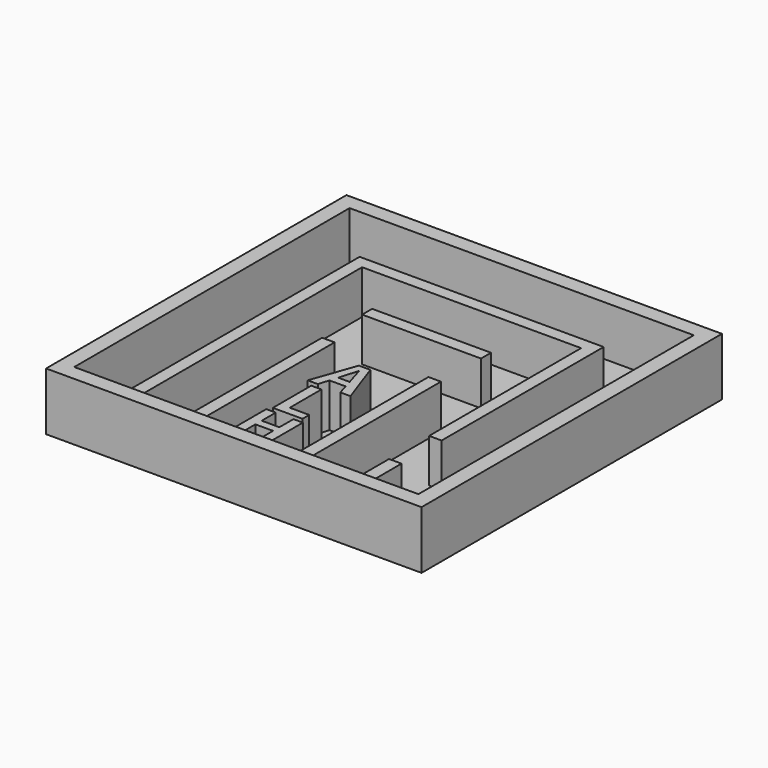
from build123d import *

# Parameters (mm, degrees)
F0_W          = 38.1
F0_H          = 38.1
F1_DEPTH      = 0.79375
F2_W          = 38.1
F2_H          = 38.1
F2_W_2        = 34.925
F2_H_2        = 34.925
F3_DEPTH      = 5.08
F4_W          = 12.065
F4_H          = 1.27
F4_W_2        = 1.27
F4_H_2        = 17.145
F4_H_3        = 4.210835259
F5_DEPTH      = 4.445
F4_R          = 1.27
F6_DEPTH      = 0.396875
F7_TEXT_SIZE  = 6.295947565
F8_DEPTH      = 4.445
F9_TEXT_SIZE  = 6.8291077494
F10_TEXT_SIZE = 6.3526599358
F11_DEPTH     = 4.445


# Not quite as in the source:
# - Text() gives the source's letters only with a copy of the font that has no kerning and outlines rounded to 1/6400 em; it was checked with that copy


with BuildPart() as f1:
    # F0 (on Top) → F1 (new body)
    with BuildSketch(Plane.XY):
        with Locations((1.3255458325, -5.1368114817)):
            Rectangle(F0_W, F0_H)
    extrude(amount=F1_DEPTH)

    # F2 (on face) → F3 (join)
    with BuildSketch(Plane.XY.offset(0.79375)):
        with Locations((1.3255458325, -5.1368114817)):
            Rectangle(F2_W, F2_H)
        with Locations((1.3255458325, -5.1368114817)):
            Rectangle(F2_W_2, F2_H_2, mode=Mode.SUBTRACT)
    extrude(amount=F3_DEPTH)

    # F4 (on face) → F5 (join)
    with BuildSketch(Plane.XY.offset(0.79375)):
        Polygon((-11.0569541675, 7.2456885183), (-11.0569541675, -22.5993114817), (-9.7869541675, -22.5993114817), (-9.7869541675, 5.9756885183), (-0.5273315559, 5.9756885183), (12.4380458325, 5.9756885183), (12.4380458325, -13.3084762228), (13.7080458325, -13.3084762228), (13.7080458325, 5.9756885183), (13.7080458325, 7.2456885183), (-9.7869541675, 7.2456885183), align=None)
        with Locations((1.3255458325, 0.2606885183)):
            Rectangle(F4_W, F4_H)
        with Locations((-4.0719541675, -14.0268114817)):
            Rectangle(F4_W_2, F4_H_2)
        with Locations((6.7230458325, -14.0268114817)):
            Rectangle(F4_W_2, F4_H_2)
        with Locations((13.0730458325, -20.4938938522)):
            Rectangle(F4_W_2, F4_H_3)
    extrude(amount=F5_DEPTH)

    # F4 (on face) → F6 (cut)
    with BuildSketch(Plane.XY.offset(0.79375)):
        with Locations((-13.5969541675, -19.2647818476)):
            Circle(F4_R)
        with Locations((-7.2469541675, -19.4972309561)):
            Circle(F4_R)
    extrude(amount=-F6_DEPTH, mode=Mode.SUBTRACT)

    # F7 (on face) → F8 (join)
    with BuildSketch(Plane.XY.offset(0.79375)):
        with Locations((-1.0268090991, -11.8785025552)):
            Text('A', F7_TEXT_SIZE, font='Open Sans', font_style=FontStyle.BOLD, text_align=(TextAlign.LEFT, TextAlign.BOTTOM))
    extrude(amount=F8_DEPTH)

    # F9 (on face) + F10 (on face) → F11 (join)
    with BuildSketch(Plane.XY.offset(0.79375)):
        with Locations((-0.848999538, -17.2861097381)):
            Text('L', F9_TEXT_SIZE, font='Open Sans', font_style=FontStyle.BOLD, text_align=(TextAlign.LEFT, TextAlign.BOTTOM))
    with BuildSketch(Plane.XY.offset(0.79375)):
        with Locations((-1.0776950512, -22.317416966)):
            Text('H', F10_TEXT_SIZE, font='Open Sans', font_style=FontStyle.BOLD, text_align=(TextAlign.LEFT, TextAlign.BOTTOM))
    extrude(amount=F11_DEPTH)


solid = f1.part
